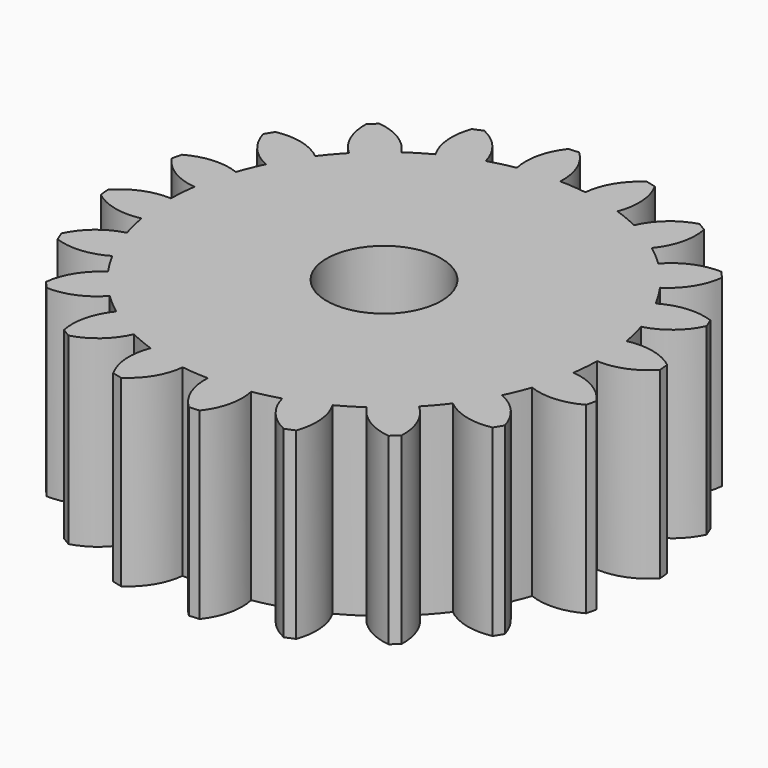
from build123d import *

# Parameters (mm, degrees)
F2_R     = 2.5
F3_DEPTH = 8


# Not quite as in the source:
# - a feature of the source that left no trace in its solid (it failed there, or was rolled back) is left out


with BuildPart() as f3:
    # F2 (on Top) → F3 (new body)
    with BuildSketch(Plane.XY):
        with BuildLine():
            ThreePointArc((-1.6229776334, 9.2680599554), (-0.7382287643, 9.3800858219), (0.1531520845, 9.4078443957))
            ThreePointArc((0.1531520845, 9.4078443957), (-0.0317997207, 10.5374998224), (-0.6817601701, 11.4797736507))
            Line((-0.6817601701, 11.4797736507), (-1.1224656787, 11.4450893749))
            ThreePointArc((-1.1224656787, 11.4450893749), (-1.6170199342, 10.4127402859), (-1.6229776334, 9.2680599554))
        make_face()
        with BuildLine():
            ThreePointArc((9.4078443957, -0.1531520845), (9.4087792756, -0.0765785786), (9.4090909091, 0))
            ThreePointArc((9.4090909091, 0), (9.3737668631, 0.8145468262), (9.2680599554, 1.6229776334))
            ThreePointArc((9.2680599554, 1.6229776334), (9.1491169783, 2.1965086508), (8.9947183137, 2.7615275108))
            ThreePointArc((8.9947183137, 2.7615275108), (8.6928665104, 3.6007032045), (8.3129211438, 4.4075314852))
            ThreePointArc((8.3129211438, 4.4075314852), (8.0225688191, 4.9162364953), (7.7011265332, 5.4058895526))
            ThreePointArc((7.7011265332, 5.4058895526), (7.1547288581, 6.1107157275), (6.5440556911, 6.7606454461))
            ThreePointArc((6.5440556911, 6.7606454461), (6.1107157275, 7.1547288581), (5.6536948308, 7.52108546))
            ThreePointArc((5.6536948308, 7.52108546), (4.9162364953, 8.0225688191), (4.1346124722, 8.4519803265))
            ThreePointArc((4.1346124722, 8.4519803265), (3.6007032045, 8.6928665104), (3.0528400867, 8.90006512))
            ThreePointArc((3.0528400867, 8.90006512), (2.1965086508, 9.1491169783), (1.320444577, 9.3159764842))
            ThreePointArc((1.320444577, 9.3159764842), (0.7382287643, 9.3800858219), (0.1531520845, 9.4078443957))
            ThreePointArc((0.1531520845, 9.4078443957), (-0.7382287643, 9.3800858219), (-1.6229776334, 9.2680599554))
            ThreePointArc((-1.6229776334, 9.2680599554), (-2.1965086508, 9.1491169783), (-2.7615275108, 8.9947183137))
            ThreePointArc((-2.7615275108, 8.9947183137), (-3.6007032045, 8.6928665104), (-4.4075314852, 8.3129211438))
            ThreePointArc((-4.4075314852, 8.3129211438), (-4.9162364953, 8.0225688191), (-5.4058895526, 7.7011265332))
            ThreePointArc((-5.4058895526, 7.7011265332), (-6.1107157275, 7.1547288581), (-6.7606454461, 6.5440556911))
            ThreePointArc((-6.7606454461, 6.5440556911), (-7.1547288581, 6.1107157275), (-7.52108546, 5.6536948308))
            ThreePointArc((-7.52108546, 5.6536948308), (-8.0225688191, 4.9162364953), (-8.4519803265, 4.1346124722))
            ThreePointArc((-8.4519803265, 4.1346124722), (-8.6928665104, 3.6007032045), (-8.90006512, 3.0528400867))
            ThreePointArc((-8.90006512, 3.0528400867), (-9.1491169783, 2.1965086508), (-9.3159764842, 1.320444577))
            ThreePointArc((-9.3159764842, 1.320444577), (-9.3800858219, 0.7382287643), (-9.4078443957, 0.1531520845))
            ThreePointArc((-9.4078443957, 0.1531520845), (-9.3800858219, -0.7382287643), (-9.2680599554, -1.6229776334))
            ThreePointArc((-9.2680599554, -1.6229776334), (-9.1491169783, -2.1965086508), (-8.9947183137, -2.7615275108))
            ThreePointArc((-8.9947183137, -2.7615275108), (-8.6928665104, -3.6007032045), (-8.3129211438, -4.4075314852))
            ThreePointArc((-8.3129211438, -4.4075314852), (-8.0225688191, -4.9162364953), (-7.7011265332, -5.4058895526))
            ThreePointArc((-7.7011265332, -5.4058895526), (-7.1547288581, -6.1107157275), (-6.5440556911, -6.7606454461))
            ThreePointArc((-6.5440556911, -6.7606454461), (-6.1107157275, -7.1547288581), (-5.6536948308, -7.52108546))
            ThreePointArc((-5.6536948308, -7.52108546), (-4.9162364953, -8.0225688191), (-4.1346124722, -8.4519803265))
            ThreePointArc((-4.1346124722, -8.4519803265), (-3.6007032045, -8.6928665104), (-3.0528400867, -8.90006512))
            ThreePointArc((-3.0528400867, -8.90006512), (-2.1965086508, -9.1491169783), (-1.320444577, -9.3159764842))
            ThreePointArc((-1.320444577, -9.3159764842), (-0.7382287643, -9.3800858219), (-0.1531520845, -9.4078443957))
            ThreePointArc((-0.1531520845, -9.4078443957), (0.7382287643, -9.3800858219), (1.6229776334, -9.2680599554))
            ThreePointArc((1.6229776334, -9.2680599554), (2.1965086508, -9.1491169783), (2.7615275108, -8.9947183137))
            ThreePointArc((2.7615275108, -8.9947183137), (3.6007032045, -8.6928665104), (4.4075314852, -8.3129211438))
            ThreePointArc((4.4075314852, -8.3129211438), (4.9162364953, -8.0225688191), (5.4058895526, -7.7011265332))
            ThreePointArc((5.4058895526, -7.7011265332), (6.1107157275, -7.1547288581), (6.7606454461, -6.5440556911))
            ThreePointArc((6.7606454461, -6.5440556911), (7.1547288581, -6.1107157275), (7.52108546, -5.6536948308))
            ThreePointArc((7.52108546, -5.6536948308), (8.0225688191, -4.9162364953), (8.4519803265, -4.1346124722))
            ThreePointArc((8.4519803265, -4.1346124722), (8.6928665104, -3.6007032045), (8.90006512, -3.0528400867))
            ThreePointArc((8.90006512, -3.0528400867), (9.1491169783, -2.1965086508), (9.3159764842, -1.320444577))
            ThreePointArc((9.3159764842, -1.320444577), (9.3800858219, -0.7382287643), (9.4078443957, -0.1531520845))
        make_face()
        Circle(F2_R, mode=Mode.SUBTRACT)
        with BuildLine():
            ThreePointArc((-4.4075314852, 8.3129211438), (-3.6007032045, 8.6928665104), (-2.7615275108, 8.9947183137))
            ThreePointArc((-2.7615275108, 8.9947183137), (-3.286509855, 10.0119312174), (-4.195837602, 10.7072380574))
            Line((-4.195837602, 10.7072380574), (-4.604255417, 10.5380658593))
            ThreePointArc((-4.604255417, 10.5380658593), (-4.7555910517, 9.4034178615), (-4.4075314852, 8.3129211438))
        make_face()
        with BuildLine():
            ThreePointArc((-6.7606454461, 6.5440556911), (-6.1107157275, 7.1547288581), (-5.4058895526, 7.7011265332))
            ThreePointArc((-5.4058895526, 7.7011265332), (-6.2195135061, 8.5063250277), (-7.2991972152, 8.8866034014))
            Line((-7.2991972152, 8.8866034014), (-7.6353485554, 8.5995030343))
            ThreePointArc((-7.6353485554, 8.5995030343), (-7.428651783, 7.4736233793), (-6.7606454461, 6.5440556911))
        make_face()
        with BuildLine():
            ThreePointArc((-8.4519803265, 4.1346124722), (-8.0225688191, 4.9162364953), (-7.52108546, 5.6536948308))
            ThreePointArc((-7.52108546, 5.6536948308), (-8.5437078414, 6.1680604771), (-9.6880605486, 6.1960860878))
            Line((-9.6880605486, 6.1960860878), (-9.9190405786, 5.8191609361))
            ThreePointArc((-9.9190405786, 5.8191609361), (-9.3745443193, 4.812258569), (-8.4519803265, 4.1346124722))
        make_face()
        with BuildLine():
            ThreePointArc((-9.3159764842, 1.320444577), (-9.1491169783, 2.1965086508), (-8.90006512, 3.0528400867))
            ThreePointArc((-8.90006512, 3.0528400867), (-10.0315845257, 3.2260231917), (-11.1285890147, 2.8990526973))
            Line((-11.1285890147, 2.8990526973), (-11.2317877999, 2.469198821))
            ThreePointArc((-11.2317877999, 2.469198821), (-10.4027911413, 1.679836361), (-9.3159764842, 1.320444577))
        make_face()
        with BuildLine():
            ThreePointArc((-9.2680599554, -1.6229776334), (-9.3800858219, -0.7382287643), (-9.4078443957, 0.1531520845))
            ThreePointArc((-9.4078443957, 0.1531520845), (-10.5374998224, -0.0317997207), (-11.4797736507, -0.6817601701))
            Line((-11.4797736507, -0.6817601701), (-11.4450893749, -1.1224656787))
            ThreePointArc((-11.4450893749, -1.1224656787), (-10.4127402859, -1.6170199342), (-9.2680599554, -1.6229776334))
        make_face()
        with BuildLine():
            ThreePointArc((-10.5380658593, -4.604255417), (-9.4034178615, -4.7555910517), (-8.3129211438, -4.4075314852))
            ThreePointArc((-8.3129211438, -4.4075314852), (-8.6928665104, -3.6007032045), (-8.9947183137, -2.7615275108))
            ThreePointArc((-8.9947183137, -2.7615275108), (-10.0119312174, -3.286509855), (-10.7072380574, -4.195837602))
            Line((-10.7072380574, -4.195837602), (-10.5380658593, -4.604255417))
        make_face()
        with BuildLine():
            ThreePointArc((-8.5995030343, -7.6353485554), (-7.4736233793, -7.428651783), (-6.5440556911, -6.7606454461))
            ThreePointArc((-6.5440556911, -6.7606454461), (-7.1547288581, -6.1107157275), (-7.7011265332, -5.4058895526))
            ThreePointArc((-7.7011265332, -5.4058895526), (-8.5063250277, -6.2195135061), (-8.8866034014, -7.2991972152))
            Line((-8.8866034014, -7.2991972152), (-8.5995030343, -7.6353485554))
        make_face()
        with BuildLine():
            ThreePointArc((-5.8191609361, -9.9190405786), (-4.812258569, -9.3745443193), (-4.1346124722, -8.4519803265))
            ThreePointArc((-4.1346124722, -8.4519803265), (-4.9162364953, -8.0225688191), (-5.6536948308, -7.52108546))
            ThreePointArc((-5.6536948308, -7.52108546), (-6.1680604771, -8.5437078414), (-6.1960860878, -9.6880605486))
            Line((-6.1960860878, -9.6880605486), (-5.8191609361, -9.9190405786))
        make_face()
        with BuildLine():
            ThreePointArc((-2.469198821, -11.2317877999), (-1.679836361, -10.4027911413), (-1.320444577, -9.3159764842))
            ThreePointArc((-1.320444577, -9.3159764842), (-2.1965086508, -9.1491169783), (-3.0528400867, -8.90006512))
            ThreePointArc((-3.0528400867, -8.90006512), (-3.2260231917, -10.0315845257), (-2.8990526973, -11.1285890147))
            Line((-2.8990526973, -11.1285890147), (-2.469198821, -11.2317877999))
        make_face()
        with BuildLine():
            ThreePointArc((1.1224656787, -11.4450893749), (1.6170199342, -10.4127402859), (1.6229776334, -9.2680599554))
            ThreePointArc((1.6229776334, -9.2680599554), (0.7382287643, -9.3800858219), (-0.1531520845, -9.4078443957))
            ThreePointArc((-0.1531520845, -9.4078443957), (0.0317997207, -10.5374998224), (0.6817601701, -11.4797736507))
            Line((0.6817601701, -11.4797736507), (1.1224656787, -11.4450893749))
        make_face()
        with BuildLine():
            ThreePointArc((4.604255417, -10.5380658593), (4.7555910517, -9.4034178615), (4.4075314852, -8.3129211438))
            ThreePointArc((4.4075314852, -8.3129211438), (3.6007032045, -8.6928665104), (2.7615275108, -8.9947183137))
            ThreePointArc((2.7615275108, -8.9947183137), (3.286509855, -10.0119312174), (4.195837602, -10.7072380574))
            Line((4.195837602, -10.7072380574), (4.604255417, -10.5380658593))
        make_face()
        with BuildLine():
            ThreePointArc((7.6353485554, -8.5995030343), (7.428651783, -7.4736233793), (6.7606454461, -6.5440556911))
            ThreePointArc((6.7606454461, -6.5440556911), (6.1107157275, -7.1547288581), (5.4058895526, -7.7011265332))
            ThreePointArc((5.4058895526, -7.7011265332), (6.2195135061, -8.5063250277), (7.2991972152, -8.8866034014))
            Line((7.2991972152, -8.8866034014), (7.6353485554, -8.5995030343))
        make_face()
        with BuildLine():
            ThreePointArc((9.9190405786, -5.8191609361), (9.3745443193, -4.812258569), (8.4519803265, -4.1346124722))
            ThreePointArc((8.4519803265, -4.1346124722), (8.0225688191, -4.9162364953), (7.52108546, -5.6536948308))
            ThreePointArc((7.52108546, -5.6536948308), (8.5437078414, -6.1680604771), (9.6880605486, -6.1960860878))
            Line((9.6880605486, -6.1960860878), (9.9190405786, -5.8191609361))
        make_face()
        with BuildLine():
            ThreePointArc((11.2317877999, -2.469198821), (10.4027911413, -1.679836361), (9.3159764842, -1.320444577))
            ThreePointArc((9.3159764842, -1.320444577), (9.1491169783, -2.1965086508), (8.90006512, -3.0528400867))
            ThreePointArc((8.90006512, -3.0528400867), (10.0315845257, -3.2260231917), (11.1285890147, -2.8990526973))
            Line((11.1285890147, -2.8990526973), (11.2317877999, -2.469198821))
        make_face()
        with BuildLine():
            ThreePointArc((9.2680599554, 1.6229776334), (9.3737668631, 0.8145468262), (9.4090909091, 0))
            ThreePointArc((9.4090909091, 0), (9.4087792756, -0.0765785786), (9.4078443957, -0.1531520845))
            ThreePointArc((9.4078443957, -0.1531520845), (10.5374998224, 0.0317997207), (11.4797736507, 0.6817601701))
            Line((11.4797736507, 0.6817601701), (11.4450893749, 1.1224656787))
            ThreePointArc((11.4450893749, 1.1224656787), (10.4127402859, 1.6170199342), (9.2680599554, 1.6229776334))
        make_face()
        with BuildLine():
            ThreePointArc((8.3129211438, 4.4075314852), (8.6928665104, 3.6007032045), (8.9947183137, 2.7615275108))
            ThreePointArc((8.9947183137, 2.7615275108), (10.0119312174, 3.286509855), (10.7072380574, 4.195837602))
            Line((10.7072380574, 4.195837602), (10.5380658593, 4.604255417))
            ThreePointArc((10.5380658593, 4.604255417), (9.4034178615, 4.7555910517), (8.3129211438, 4.4075314852))
        make_face()
        with BuildLine():
            ThreePointArc((6.5440556911, 6.7606454461), (7.1547288581, 6.1107157275), (7.7011265332, 5.4058895526))
            ThreePointArc((7.7011265332, 5.4058895526), (8.5063250277, 6.2195135061), (8.8866034014, 7.2991972152))
            Line((8.8866034014, 7.2991972152), (8.5995030343, 7.6353485554))
            ThreePointArc((8.5995030343, 7.6353485554), (7.4736233793, 7.428651783), (6.5440556911, 6.7606454461))
        make_face()
        with BuildLine():
            ThreePointArc((4.1346124722, 8.4519803265), (4.9162364953, 8.0225688191), (5.6536948308, 7.52108546))
            ThreePointArc((5.6536948308, 7.52108546), (6.1680604771, 8.5437078414), (6.1960860878, 9.6880605486))
            Line((6.1960860878, 9.6880605486), (5.8191609361, 9.9190405786))
            ThreePointArc((5.8191609361, 9.9190405786), (4.812258569, 9.3745443193), (4.1346124722, 8.4519803265))
        make_face()
        with BuildLine():
            ThreePointArc((1.320444577, 9.3159764842), (2.1965086508, 9.1491169783), (3.0528400867, 8.90006512))
            ThreePointArc((3.0528400867, 8.90006512), (3.2260231917, 10.0315845257), (2.8990526973, 11.1285890147))
            Line((2.8990526973, 11.1285890147), (2.469198821, 11.2317877999))
            ThreePointArc((2.469198821, 11.2317877999), (1.679836361, 10.4027911413), (1.320444577, 9.3159764842))
        make_face()
    extrude(amount=F3_DEPTH)


solid = f3.part
